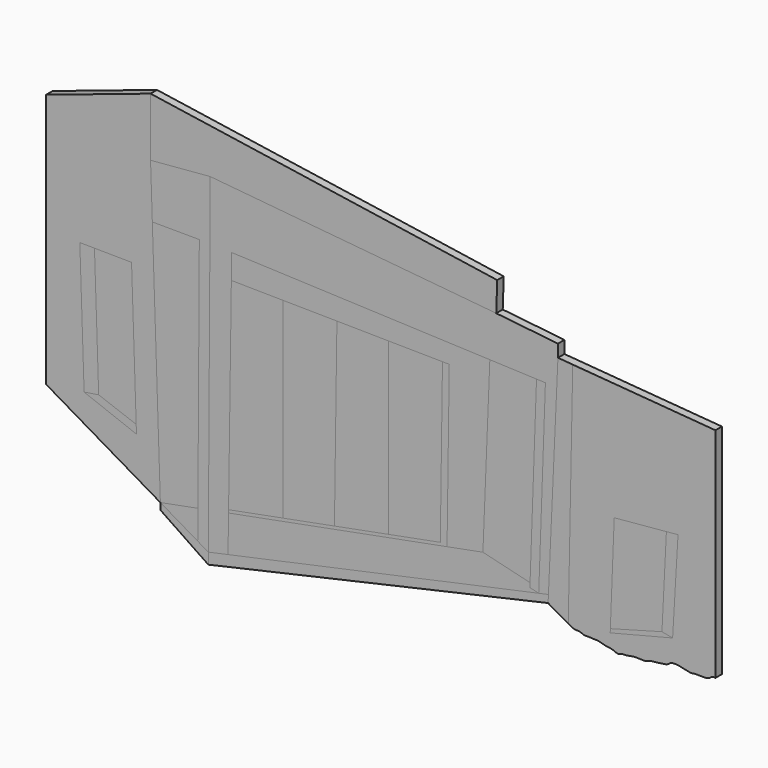
from build123d import *

# Parameters (mm, degrees)
F2_DEPTH  = 2.54
F3_DEPTH  = 2.54
F4_DEPTH  = 2.54
F5_DEPTH  = 2.54
F6_DEPTH  = 2.54
F7_DEPTH  = 2.54
F8_DEPTH  = 2.54
F9_DEPTH  = 2.54
F10_DEPTH = 2.54
F11_DEPTH = 2.54
F12_DEPTH = 2.54
F13_DEPTH = 2.54
F14_DEPTH = 2.54
F15_DEPTH = 2.54
F16_DEPTH = 2.54
F17_DEPTH = 2.54
F18_DEPTH = 2.54
F19_DEPTH = 2.54
F20_DEPTH = 2.54
F21_DEPTH = 2.54
F22_DEPTH = 2.54
F23_DEPTH = 2.54


with BuildPart() as f2:
    # F1 (on Front) → F2 (new body)
    with BuildSketch(Plane.XZ):
        Polygon((-74.0562155843, 73.7754032016), (-106.7237751558, 62.8445893526), (-106.7237751558, -16.8648809195), (-70.9872841835, -37.785153836), (-73.503443121, 38.6428111936), (-74.0562155843, 55.4331950843), align=None)
        Polygon((-91.5920581143, 25.533032684), (-79.9994021654, 25.4001282156), (-78.5467419713, -18.7242157825), (-78.4587935546, -21.395636262), (-94.8317199945, -15.1276020333), (-96.1720767265, 25.5855404908), align=None, mode=Mode.SUBTRACT)
    extrude(amount=F2_DEPTH)


with BuildPart() as f3:
    # F1 (on Front) → F3 (new body)
    with BuildSketch(Plane.XZ):
        Polygon((34.352902323, 57.6994121075), (-74.0562155843, 73.7754032016), (-74.0562155843, 55.4331950843), (-55.3896278143, 57.0179112256), (34.0380035341, 48.4676808119), align=None)
    extrude(amount=F3_DEPTH)


with BuildPart() as f4:
    # F1 (on Front) → F4 (new body)
    with BuildSketch(Plane.XZ):
        with BuildLine():
            Line((102.5799615309, -29.6344310045), (102.5799615309, 38.5525114834))
            Line((102.5799615309, 38.5525114834), (57.9592958093, 41.9228598475))
            Line((57.9592958093, 41.9228598475), (56.5582178533, -29.6344310045))
            add(Edge.make_bspline(
                [(56.5582178533, -29.6344310045), (57.2856265627, -30.0462591399), (58.5941860457, -30.7871103353), (60.082729297, -30.4653642105), (61.4709755846, -31.321777245), (62.0915416084, -31.1476431787), (63.6574457486, -31.2564378868), (64.8604179511, -31.3261618759), (66.1358190748, -31.2493937435), (67.9914564947, -32.0184292859), (70.5972844991, -32.1477207339), (72.0214962613, -33.1579149882), (73.5307889186, -32.4239339531), (74.2079501693, -32.5971585772), (76.7310536587, -32.1041454845), (77.3853124381, -32.0519940362), (78.4703855183, -32.0348592947), (80.3479498378, -32.1743745067), (80.8859972848, -32.0763453371), (81.5510971492, -31.8648744104), (82.3848678505, -31.3744772884), (87.5481842057, -31.1235127629), (88.0682910334, -30.3074440344), (88.9242772648, -29.9073784324), (89.3529124413, -29.8977596483), (90.9450907289, -29.7805471371), (94.9396023411, -30.9419191035), (95.9169789936, -30.5329169819), (98.0284682793, -30.6408599128), (99.4940083351, -30.6199291335), (100.8535584753, -30.3333131266), (101.5166423935, -29.4679385788), (102.2238121812, -29.5786658376), (102.5799615309, -29.6344310045)],
                knots=[0, 0, 0, 0, 0.0412321749, 0.0741739173, 0.1069894815, 0.1285274588, 0.1620195505, 0.1924920609, 0.2223241885, 0.2608161073, 0.3047766154, 0.3395638668, 0.3718264529, 0.3957989152, 0.4385152033, 0.4613675493, 0.48952259, 0.5268741309, 0.5472124496, 0.5680019419, 0.595893804, 0.6565254336, 0.6832286331, 0.7078270845, 0.7249293991, 0.7589934478, 0.8140591093, 0.8426155771, 0.8809427666, 0.9150067343, 0.9460941279, 0.9728515816, 1, 1, 1, 1], degree=3))
        make_face()
        Polygon((69.7227070782, -26.7481742461), (70.9294527769, 4.1724690236), (87.2491845391, 5.6631790631), (90.8821895719, 5.9950323775), (89.1989469528, -22.9926872998), (69.6771070361, -27.9165916145), align=None, mode=Mode.SUBTRACT)
    extrude(amount=F4_DEPTH)


with BuildPart() as f5:
    # F1 (on Front) → F5 (new body)
    with BuildSketch(Plane.XZ):
        Polygon((-73.503443121, 38.6428111936), (-70.9872841835, -37.785153836), (-59.2448789076, -35.5592972244), (-58.8094183001, 38.5564777649), align=None)
    extrude(amount=F5_DEPTH)


with BuildPart() as f5b:
    # F1 (on Front) → F5, piece 2 (new body)
    with BuildSketch(Plane.XZ):
        Polygon((29.8768132925, -18.6656452715), (32.0387599567, 35.0360945784), (-48.6874692142, 38.2860042155), (-48.7928533968, 30.568183665), (-32.6999797354, 30.3484410155), (-15.7811137564, 30.1174197252), (0.3224367358, 29.8975312871), (17.230625884, 29.6666557853), (19.3502480039, 29.637713075), (18.6616536589, -20.7915587138), align=None)
    extrude(amount=F5_DEPTH)


with BuildPart() as f6:
    # F1 (on Front) → F6 (new body)
    with BuildSketch(Plane.XZ):
        Polygon((-55.3896278143, 57.0179112256), (-74.0562155843, 55.4331950843), (-73.503443121, 38.6428111936), (-58.8094183001, 38.5564777649), (-59.2448789076, -35.5592972244), (-59.298161314, -44.628009246), (-55.9981895392, -46.5598248292), (-55.4982106199, 38.5370230603), align=None)
    extrude(amount=F6_DEPTH)


with BuildPart() as f7:
    # F1 (on Front) → F7 (new body)
    with BuildSketch(Plane.XZ):
        Polygon((50.3595485047, -23.6380400372), (53.3372536302, 42.4973480403), (53.3372536302, 46.388220042), (34.0380035341, 48.4676808119), (-55.3896278143, 57.0179112256), (-55.4982106199, 38.5370230603), (-55.9981895392, -46.5598248292), (-49.8246848583, -45.2293363446), (-49.8246848583, -44.9980907142), (-49.6710210091, -33.7445042241), (-49.6585152161, -32.8286412977), (-48.7928533968, 30.568183665), (-48.6874692142, 38.2860042155), (32.0387599567, 35.0360945784), (46.6352587909, 34.4484627428), (49.4159013033, 34.3365184963), (47.3254715631, -24.2919318929), align=None)
    extrude(amount=F7_DEPTH)


with BuildPart() as f8:
    # F1 (on Front) → F8 (new body)
    with BuildSketch(Plane.XZ):
        Polygon((56.5582178533, -29.6344310045), (57.9592958093, 41.9228598475), (53.3372536302, 42.4973480403), (50.3595485047, -23.6380400372), (50.2515248954, -26.0372646153), align=None)
    extrude(amount=F8_DEPTH)


with BuildPart() as f8b:
    # F1 (on Front) → F8, piece 2 (new body)
    with BuildSketch(Plane.XZ):
        Polygon((44.6138855261, -22.2432212191), (46.6352587909, 34.4484627428), (32.0387599567, 35.0360945784), (29.8768132925, -18.6656452715), align=None)
    extrude(amount=F8_DEPTH)


with BuildPart() as f9:
    # F1 (on Front) → F9 (new body)
    with BuildSketch(Plane.XZ):
        Polygon((44.5647338779, -23.6217344084), (47.3254715631, -24.2919318929), (49.4159013033, 34.3365184963), (46.6352587909, 34.4484627428), (44.6138855261, -22.2432212191), align=None)
    extrude(amount=F9_DEPTH)


with BuildPart() as f10:
    # F1 (on Front) → F10 (new body)
    with BuildSketch(Plane.XZ):
        Polygon((-59.2448789076, -35.5592972244), (-70.9872841835, -37.785153836), (-59.298161314, -44.628009246), align=None)
    extrude(amount=F10_DEPTH)


with BuildPart() as f10b:
    # F1 (on Front) → F10, piece 2 (new body)
    with BuildSketch(Plane.XZ):
        Polygon((-49.8246848583, -45.2293363446), (47.3254715631, -24.2919318929), (44.5647338779, -23.6217344084), (44.6138855261, -22.2432212191), (29.8768132925, -18.6656452715), (18.6616536589, -20.7915587138), (-49.6710210091, -33.7445042241), (-49.8246848583, -44.9980907142), align=None)
    extrude(amount=F10_DEPTH)


with BuildPart() as f11:
    # F1 (on Front) → F11 (new body)
    with BuildSketch(Plane.XZ):
        Polygon((-59.298161314, -44.628009246), (-70.9872841835, -37.785153836), (-70.9872841835, -39.8426502943), (-55.9981895392, -50.0132987777), (-55.9981895392, -46.5598248292), align=None)
    extrude(amount=F11_DEPTH)


with BuildPart() as f12:
    # F1 (on Front) → F12 (new body)
    with BuildSketch(Plane.XZ):
        Polygon((50.2515248954, -26.0372646153), (50.3595485047, -23.6380400372), (47.3254715631, -24.2919318929), (-49.8246848583, -45.2293363446), (-55.9981895392, -46.5598248292), (-55.9981895392, -50.0132987777), (-51.7402192231, -49.0524562728), align=None)
    extrude(amount=F12_DEPTH)


with BuildPart() as f13:
    # F1 (on Front) → F13 (new body)
    with BuildSketch(Plane.XZ):
        Polygon((16.5486405693, -20.2786030408), (18.6616536589, -20.7915587138), (19.3502480039, 29.637713075), (17.230625884, 29.6666557853), align=None)
        Polygon((-49.6585152161, -32.8286412977), (-49.6710210091, -33.7445042241), (18.6616536589, -20.7915587138), (16.5486405693, -20.2786030408), (0.3224367358, -23.3543956263), (-16.5549373234, -26.5536221692), (-32.6999797354, -29.6140300289), align=None)
    extrude(amount=F13_DEPTH)


with BuildPart() as f14:
    # F1 (on Front) → F14 (new body)
    with BuildSketch(Plane.XZ):
        Polygon((-48.7928533968, 30.568183665), (-49.6585152161, -32.8286412977), (-32.6999797354, -29.6140300289), (-32.6999797354, 0.0969890625), (-32.6999797354, 30.3484410155), align=None)
    extrude(amount=F14_DEPTH)


with BuildPart() as f15:
    # F1 (on Front) → F15 (new body)
    with BuildSketch(Plane.XZ):
        Polygon((-32.6999797354, 0.0969890625), (-32.6999797354, -29.6140300289), (-16.5549373234, -26.5536221692), (-15.7813113578, 30.10294837), (-15.7811137564, 30.1174197252), (-32.6999797354, 30.3484410155), align=None)
    extrude(amount=F15_DEPTH)


with BuildPart() as f16:
    # F1 (on Front) → F16 (new body)
    with BuildSketch(Plane.XZ):
        Polygon((-15.7813113578, 30.10294837), (-16.5549373234, -26.5536221692), (0.3224367358, -23.3543956263), (0.3224367358, 29.8975312871), (-15.7811137564, 30.1174197252), align=None)
    extrude(amount=F16_DEPTH)


with BuildPart() as f17:
    # F1 (on Front) → F17 (new body)
    with BuildSketch(Plane.XZ):
        Polygon((0.3224367358, -23.3543956263), (16.5486405693, -20.2786030408), (17.230625884, 29.6666557853), (0.3224367358, 29.8975312871), align=None)
    extrude(amount=F17_DEPTH)


with BuildPart() as f18:
    # F1 (on Front) → F18 (new body)
    with BuildSketch(Plane.XZ):
        Polygon((-90.2769300282, -14.4137933567), (-91.5920581143, 25.533032684), (-96.1720767265, 25.5855404908), (-94.8317199945, -15.1276020333), align=None)
    extrude(amount=F18_DEPTH)


with BuildPart() as f19:
    # F1 (on Front) → F19 (new body)
    with BuildSketch(Plane.XZ):
        Polygon((-78.4587935546, -21.395636262), (-78.5467419713, -18.7242157825), (-90.2769300282, -14.4137933567), (-94.8317199945, -15.1276020333), align=None)
    extrude(amount=F19_DEPTH)


with BuildPart() as f20:
    # F1 (on Front) → F20 (new body)
    with BuildSketch(Plane.XZ):
        Polygon((90.8821895719, 5.9950323775), (87.2491845391, 5.6631790631), (87.238651334, 5.4513658579), (85.8566118794, -22.3401946629), (89.1989469528, -22.9926872998), align=None)
    extrude(amount=F20_DEPTH)


with BuildPart() as f21:
    # F1 (on Front) → F21 (new body)
    with BuildSketch(Plane.XZ):
        Polygon((85.8566118794, -22.3401946628), (69.7227070782, -26.7481742461), (69.6771070361, -27.9165916145), (89.1989469528, -22.9926872998), align=None)
    extrude(amount=F21_DEPTH)


with BuildPart() as f22:
    # F1 (on Front) → F22 (new body)
    with BuildSketch(Plane.XZ):
        Polygon((-78.5467419713, -18.7242157825), (-79.9994021654, 25.4001282156), (-91.5920581143, 25.533032684), (-90.2769300282, -14.4137933567), align=None)
    extrude(amount=F22_DEPTH)


with BuildPart() as f22b:
    # F1 (on Front) → F22, piece 2 (new body)
    with BuildSketch(Plane.XZ):
        Polygon((87.2491845391, 5.6631790631), (70.9294527769, 4.1724690236), (69.7227070782, -26.7481742461), (85.8566118794, -22.3401946628), (87.238651334, 5.4513658579), align=None)
    extrude(amount=F22_DEPTH)


with BuildPart() as f23:
    # F1 (on Front) → F23 (new body)
    with BuildSketch(Plane.XZ):
        Polygon((57.9592958093, 41.9228598475), (102.5799615309, 38.5525114834), (53.3372536302, 42.4973480403), align=None)
    extrude(amount=F23_DEPTH)


solid = Compound([f2.part, f3.part, f4.part, f5.part, f5b.part, f6.part, f7.part, f8.part, f8b.part, f9.part, f10.part, f10b.part, f11.part, f12.part, f13.part, f14.part, f15.part, f16.part, f17.part, f18.part, f19.part, f20.part, f21.part, f22.part, f22b.part, f23.part])
